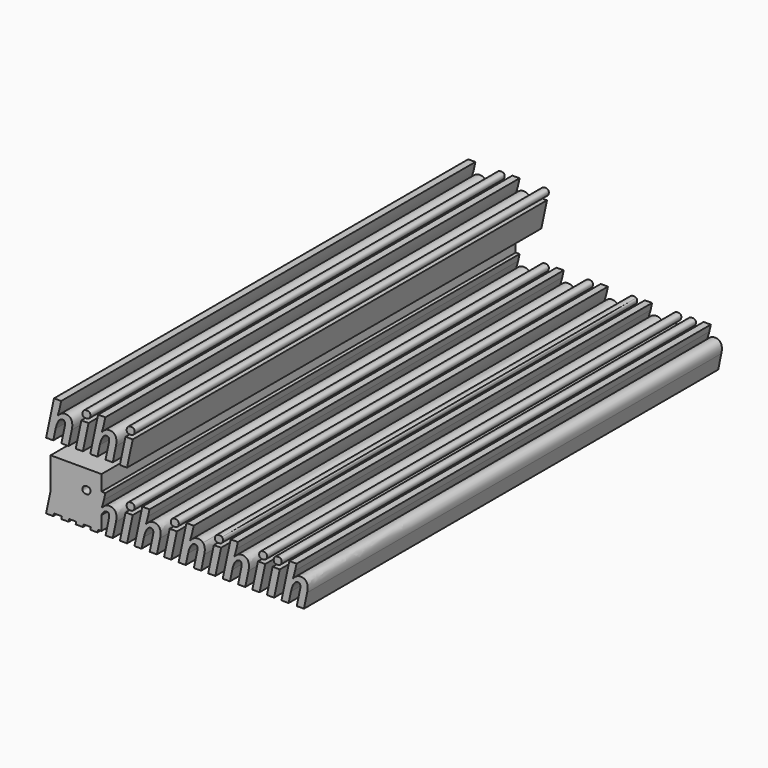
from build123d import *

# Parameters (mm, degrees)
F0_TEXT_SIZE = 47.1805429293
F1_DEPTH     = 498.348


# Not quite as in the source:
# - Text() gives the source's letters only with a copy of the font that has no kerning and outlines rounded to 1/6400 em; it was checked with that copy


with BuildPart() as f1:
    # F0 (on Front) → F1 (new body)
    with BuildSketch(Plane.XZ):
        with BuildLine():
            Line((7.1037112932, -24.0933876485), (14.1806185259, -24.0933876485))
            Line((14.1806185259, -24.0933876485), (21.2442852385, 9.2243729952))
            Line((21.2442852385, 9.2243729952), (24.4913287461, 9.2243729952))
            Line((24.4913287461, 9.2243729952), (24.4913287461, 24.0933876485))
            Line((24.4913287461, 24.0933876485), (-24.4913287461, 24.0933876485))
            Line((-24.4913287461, 24.0933876485), (-24.4913287461, -6.005607145))
            Line((-24.4913287461, -6.005607145), (-21.2624351568, 9.2243729952))
            Line((-21.2624351568, 9.2243729952), (-14.3254209543, 9.2243729952))
            add(Edge.make_bspline(
                [(-14.3254209543, 9.2243729952), (-15.2248000539, 5.0518437298), (-15.7113494028, 2.8181399005)],
                knots=[0, 0, 0, 1, 1, 1], degree=2))
            add(Edge.make_bspline(
                [(-15.7113494028, 2.8181399005), (-16.1978987518, 0.5844360712), (-17.6944065978, -4.3031732979)],
                knots=[0, 0, 0, 1, 1, 1], degree=2))
            Line((-17.6944065978, -4.3031732979), (-17.510107602, -4.3031732979))
            add(Edge.make_bspline(
                [(-17.510107602, -4.3031732979), (-16.0799473944, -2.5265309782), (-14.3291069342, -1.4575968024)],
                knots=[0, 0, 0, 1, 1, 1], degree=2))
            add(Edge.make_bspline(
                [(-14.3291069342, -1.4575968024), (-12.5782664739, -0.3886626267), (-10.2708430463, -0.3886626267)],
                knots=[0, 0, 0, 1, 1, 1], degree=2))
            add(Edge.make_bspline(
                [(-10.2708430463, -0.3886626267), (-7.0935283584, -0.3886626267), (-5.3537458379, -2.3090581631)],
                knots=[0, 0, 0, 1, 1, 1], degree=2))
            add(Edge.make_bspline(
                [(-5.3537458379, -2.3090581631), (-3.6139633173, -4.2294536995), (-3.6139633173, -7.8048542184)],
                knots=[0, 0, 0, 1, 1, 1], degree=2))
            add(Edge.make_bspline(
                [(-3.6139633173, -7.8048542184), (-3.6139633173, -9.4856610603), (-4.1447444253, -11.9478956444)],
                knots=[0, 0, 0, 1, 1, 1], degree=2))
            Line((-4.1447444253, -11.9478956444), (-6.6824263307, -24.0933876485))
            Line((-6.6824263307, -24.0933876485), (0.1733443567, -24.0933876485))
            Line((0.1733443567, -24.0933876485), (5.0923212451, -0.8678400158))
            Line((5.0923212451, -0.8678400158), (12.0293354477, -0.8678400158))
            Line((12.0293354477, -0.8678400158), (7.1037112932, -24.0933876485))
        make_face()
        with BuildLine():
            add(Edge.make_bspline(
                [(9.677680261, 2.3315905516), (6.19811522, 2.3315905516), (6.19811522, 5.1697950872)],
                knots=[0, 0, 0, 1, 1, 1], degree=2))
            add(Edge.make_bspline(
                [(6.19811522, 5.1697950872), (6.19811522, 7.1675962018), (7.2928512551, 8.1959845985)],
                knots=[0, 0, 0, 1, 1, 1], degree=2))
            add(Edge.make_bspline(
                [(7.2928512551, 8.1959845985), (8.3875872903, 9.2243729952), (10.3927603648, 9.2243729952)],
                knots=[0, 0, 0, 1, 1, 1], degree=2))
            add(Edge.make_bspline(
                [(10.3927603648, 9.2243729952), (12.0735672066, 9.2243729952), (12.9508304267, 8.5092928914)],
                knots=[0, 0, 0, 1, 1, 1], degree=2))
            add(Edge.make_bspline(
                [(12.9508304267, 8.5092928914), (13.8280936468, 7.7942127876), (13.8280936468, 6.4598880579)],
                knots=[0, 0, 0, 1, 1, 1], degree=2))
            add(Edge.make_bspline(
                [(13.8280936468, 6.4598880579), (13.8280936468, 4.6168980997), (12.8144491698, 3.4742443256)],
                knots=[0, 0, 0, 1, 1, 1], degree=2))
            add(Edge.make_bspline(
                [(12.8144491698, 3.4742443256), (11.8008046928, 2.3315905516), (9.677680261, 2.3315905516)],
                knots=[0, 0, 0, 1, 1, 1], degree=2))
        make_face(mode=Mode.SUBTRACT)
        with BuildLine():
            Line((21.1106508309, -24.0933876485), (24.4913287461, -24.0933876485))
            Line((24.4913287461, -24.0933876485), (24.4913287461, -10.5974846616))
            add(Edge.make_bspline(
                [(24.4913287461, -10.5974846616), (23.4979536486, -12.8144800029), (22.8366285624, -15.9582417934)],
                knots=[0.3305359837, 0.3305359837, 0.3305359837, 1, 1, 1], degree=2))
            Line((22.8366285624, -15.9582417934), (21.1106508309, -24.0933876485))
        make_face()
        Polygon((20.5734368938, -26.6254676713), (21.1106508309, -24.0933876485), (14.1806185259, -24.0933876485), (13.643794651, -26.6254676713), align=None)
        with BuildLine():
            Line((14.1806185259, -24.0933876485), (21.1106508309, -24.0933876485))
            Line((21.1106508309, -24.0933876485), (22.8366285624, -15.9582417934))
            add(Edge.make_bspline(
                [(24.4913287461, -10.5974846616), (23.4979536486, -12.8144800029), (22.8366285624, -15.9582417934)],
                knots=[0.3305359837, 0.3305359837, 0.3305359837, 1, 1, 1], degree=2))
            Line((24.4913287461, -10.5974846616), (24.4913287461, 9.2243729952))
            Line((24.4913287461, 9.2243729952), (21.2442852385, 9.2243729952))
            Line((21.2442852385, 9.2243729952), (14.1806185259, -24.0933876485))
        make_face()
        with BuildLine():
            Line((24.4913287461, 9.2243729952), (24.4913287461, -10.5974846616))
            add(Edge.make_bspline(
                [(25.5531957607, -8.6341996996), (24.9817900809, -9.5028825349), (24.4913287461, -10.5974846616)],
                knots=[0, 0, 0, 0.3305359837, 0.3305359837, 0.3305359837], degree=2))
            add(Edge.make_bspline(
                [(29.3976728135, -6.0060960192), (27.2819203415, -6.0060960192), (25.5531957607, -8.6341996996)],
                knots=[0, 0, 0, 1, 1, 1], degree=2))
            add(Edge.make_bspline(
                [(31.889395237, -8.836928595), (31.889395237, -6.0060960192), (29.3976728135, -6.0060960192)],
                knots=[0, 0, 0, 1, 1, 1], degree=2))
            add(Edge.make_bspline(
                [(31.5207972453, -11.5792976527), (31.889395237, -10.0164421682), (31.889395237, -8.836928595)],
                knots=[0, 0, 0, 1, 1, 1], degree=2))
            Line((31.5207972453, -11.5792976527), (28.3655984369, -26.6254676713))
            Line((28.3655984369, -26.6254676713), (35.2952406797, -26.6254676713))
            Line((35.2952406797, -26.6254676713), (38.3619759701, -11.9478956444))
            add(Edge.make_bspline(
                [(38.892757078, -7.8048542184), (38.892757078, -9.4856610603), (38.3619759701, -11.9478956444)],
                knots=[0, 0, 0, 1, 1, 1], degree=2))
            add(Edge.make_bspline(
                [(37.1529745575, -2.3090581631), (38.892757078, -4.2294536995), (38.892757078, -7.8048542184)],
                knots=[0, 0, 0, 1, 1, 1], degree=2))
            add(Edge.make_bspline(
                [(32.2358773491, -0.3886626267), (35.413192037, -0.3886626267), (37.1529745575, -2.3090581631)],
                knots=[0, 0, 0, 1, 1, 1], degree=2))
            add(Edge.make_bspline(
                [(28.1776134612, -1.4575968024), (29.9284539215, -0.3886626267), (32.2358773491, -0.3886626267)],
                knots=[0, 0, 0, 1, 1, 1], degree=2))
            add(Edge.make_bspline(
                [(24.9966127934, -4.3031732979), (26.4267730009, -2.5265309782), (28.1776134612, -1.4575968024)],
                knots=[0, 0, 0, 1, 1, 1], degree=2))
            Line((24.9966127934, -4.3031732979), (24.8123137976, -4.3031732979))
            add(Edge.make_bspline(
                [(26.7953709926, 2.8181399005), (26.3088216436, 0.5844360712), (24.8123137976, -4.3031732979)],
                knots=[0, 0, 0, 1, 1, 1], degree=2))
            add(Edge.make_bspline(
                [(28.1812994411, 9.2243729952), (27.2819203415, 5.0518437298), (26.7953709926, 2.8181399005)],
                knots=[0, 0, 0, 1, 1, 1], degree=2))
            Line((28.1812994411, 9.2243729952), (24.4913287461, 9.2243729952))
        make_face()
        Polygon((6.5667132116, -26.6254676713), (7.1037112932, -24.0933876485), (0.1733443567, -24.0933876485), (-0.3629290311, -26.6254676713), align=None)
        Polygon((0.1733443567, -24.0933876485), (7.1037112932, -24.0933876485), (12.0293354477, -0.8678400158), (5.0923212451, -0.8678400158), align=None)
        Polygon((-7.2114797157, -26.6254676713), (-6.6824263307, -24.0933876485), (-13.6101419243, -24.0933876485), (-14.1411219584, -26.6254676713), align=None)
        with BuildLine():
            Line((-13.6101419243, -24.0933876485), (-6.6824263307, -24.0933876485))
            Line((-6.6824263307, -24.0933876485), (-4.1447444253, -11.9478956444))
            add(Edge.make_bspline(
                [(-3.6139633173, -7.8048542184), (-3.6139633173, -9.4856610603), (-4.1447444253, -11.9478956444)],
                knots=[0, 0, 0, 1, 1, 1], degree=2))
            add(Edge.make_bspline(
                [(-5.3537458379, -2.3090581631), (-3.6139633173, -4.2294536995), (-3.6139633173, -7.8048542184)],
                knots=[0, 0, 0, 1, 1, 1], degree=2))
            add(Edge.make_bspline(
                [(-10.2708430463, -0.3886626267), (-7.0935283584, -0.3886626267), (-5.3537458379, -2.3090581631)],
                knots=[0, 0, 0, 1, 1, 1], degree=2))
            add(Edge.make_bspline(
                [(-14.3291069342, -1.4575968024), (-12.5782664739, -0.3886626267), (-10.2708430463, -0.3886626267)],
                knots=[0, 0, 0, 1, 1, 1], degree=2))
            add(Edge.make_bspline(
                [(-17.510107602, -4.3031732979), (-16.0799473944, -2.5265309782), (-14.3291069342, -1.4575968024)],
                knots=[0, 0, 0, 1, 1, 1], degree=2))
            Line((-17.510107602, -4.3031732979), (-17.6944065978, -4.3031732979))
            add(Edge.make_bspline(
                [(-15.7113494028, 2.8181399005), (-16.1978987518, 0.5844360712), (-17.6944065978, -4.3031732979)],
                knots=[0, 0, 0, 1, 1, 1], degree=2))
            add(Edge.make_bspline(
                [(-14.3254209543, 9.2243729952), (-15.2248000539, 5.0518437298), (-15.7113494028, 2.8181399005)],
                knots=[0, 0, 0, 1, 1, 1], degree=2))
            Line((-14.3254209543, 9.2243729952), (-21.2624351568, 9.2243729952))
            Line((-21.2624351568, 9.2243729952), (-24.4913287461, -6.005607145))
            Line((-24.4913287461, -6.005607145), (-24.4913287461, -24.0933876485))
            Line((-24.4913287461, -24.0933876485), (-21.3960695645, -24.0933876485))
            Line((-21.3960695645, -24.0933876485), (-19.670091833, -15.9582417934))
            add(Edge.make_bspline(
                [(-16.9535246346, -8.6341996996), (-18.6822492154, -11.2623033799), (-19.670091833, -15.9582417934)],
                knots=[0, 0, 0, 1, 1, 1], degree=2))
            add(Edge.make_bspline(
                [(-13.1090475819, -6.0060960192), (-15.2248000539, -6.0060960192), (-16.9535246346, -8.6341996996)],
                knots=[0, 0, 0, 1, 1, 1], degree=2))
            add(Edge.make_bspline(
                [(-10.6173251584, -8.836928595), (-10.6173251584, -6.0060960192), (-13.1090475819, -6.0060960192)],
                knots=[0, 0, 0, 1, 1, 1], degree=2))
            add(Edge.make_bspline(
                [(-10.98592315, -11.5792976527), (-10.6173251584, -10.0164421682), (-10.6173251584, -8.836928595)],
                knots=[0, 0, 0, 1, 1, 1], degree=2))
            Line((-10.98592315, -11.5792976527), (-13.6101419243, -24.0933876485))
        make_face()
        Polygon((-24.4913287461, -24.0933876485), (-24.4913287461, -6.005607145), (-28.8629257444, -26.6254676713), (-21.9332835016, -26.6254676713), (-21.3960695645, -24.0933876485), align=None)
        with BuildLine():
            Line((-21.3960695645, -24.0933876485), (-13.6101419243, -24.0933876485))
            Line((-13.6101419243, -24.0933876485), (-10.98592315, -11.5792976527))
            add(Edge.make_bspline(
                [(-10.98592315, -11.5792976527), (-10.6173251584, -10.0164421682), (-10.6173251584, -8.836928595)],
                knots=[0, 0, 0, 1, 1, 1], degree=2))
            add(Edge.make_bspline(
                [(-10.6173251584, -8.836928595), (-10.6173251584, -6.0060960192), (-13.1090475819, -6.0060960192)],
                knots=[0, 0, 0, 1, 1, 1], degree=2))
            add(Edge.make_bspline(
                [(-13.1090475819, -6.0060960192), (-15.2248000539, -6.0060960192), (-16.9535246346, -8.6341996996)],
                knots=[0, 0, 0, 1, 1, 1], degree=2))
            add(Edge.make_bspline(
                [(-16.9535246346, -8.6341996996), (-18.6822492154, -11.2623033799), (-19.670091833, -15.9582417934)],
                knots=[0, 0, 0, 1, 1, 1], degree=2))
            Line((-19.670091833, -15.9582417934), (-21.3960695645, -24.0933876485))
        make_face()
        with Locations((-29.718073085, 37.5400707126)):
            Text('hihi', F0_TEXT_SIZE, font='Open Sans', font_style=FontStyle.BOLDITALIC, text_align=(TextAlign.LEFT, TextAlign.BOTTOM))
        with BuildLine():
            add(Edge.make_bspline(
                [(48.7048356154, 5.1697950872), (48.7048356154, 7.1675962018), (49.7995716505, 8.1959845985)],
                knots=[0, 0, 0, 1, 1, 1], degree=2))
            add(Edge.make_bspline(
                [(52.1844006564, 2.3315905516), (48.7048356154, 2.3315905516), (48.7048356154, 5.1697950872)],
                knots=[0, 0, 0, 1, 1, 1], degree=2))
            add(Edge.make_bspline(
                [(55.3211695652, 3.4742443256), (54.3075250882, 2.3315905516), (52.1844006564, 2.3315905516)],
                knots=[0, 0, 0, 1, 1, 1], degree=2))
            add(Edge.make_bspline(
                [(56.3348140422, 6.4598880579), (56.3348140422, 4.6168980997), (55.3211695652, 3.4742443256)],
                knots=[0, 0, 0, 1, 1, 1], degree=2))
            add(Edge.make_bspline(
                [(55.4575508221, 8.5092928914), (56.3348140422, 7.7942127876), (56.3348140422, 6.4598880579)],
                knots=[0, 0, 0, 1, 1, 1], degree=2))
            add(Edge.make_bspline(
                [(52.8994807602, 9.2243729952), (54.580287602, 9.2243729952), (55.4575508221, 8.5092928914)],
                knots=[0, 0, 0, 1, 1, 1], degree=2))
            add(Edge.make_bspline(
                [(49.7995716505, 8.1959845985), (50.8943076857, 9.2243729952), (52.8994807602, 9.2243729952)],
                knots=[0, 0, 0, 1, 1, 1], degree=2))
        make_face()
        Polygon((42.1437913642, -26.6254676713), (49.073433607, -26.6254676713), (54.536055843, -0.8678400158), (47.5990416404, -0.8678400158), align=None)
        with BuildLine():
            Line((70.8723188323, -26.6254676713), (77.801961075, -26.6254676713))
            Line((77.801961075, -26.6254676713), (80.8686963654, -11.9478956444))
            add(Edge.make_bspline(
                [(81.3994774734, -7.8048542184), (81.3994774734, -9.4856610603), (80.8686963654, -11.9478956444)],
                knots=[0, 0, 0, 1, 1, 1], degree=2))
            add(Edge.make_bspline(
                [(79.6596949529, -2.3090581631), (81.3994774734, -4.2294536995), (81.3994774734, -7.8048542184)],
                knots=[0, 0, 0, 1, 1, 1], degree=2))
            add(Edge.make_bspline(
                [(74.7425977445, -0.3886626267), (77.9199124324, -0.3886626267), (79.6596949529, -2.3090581631)],
                knots=[0, 0, 0, 1, 1, 1], degree=2))
            add(Edge.make_bspline(
                [(70.6843338566, -1.4575968024), (72.4351743168, -0.3886626267), (74.7425977445, -0.3886626267)],
                knots=[0, 0, 0, 1, 1, 1], degree=2))
            add(Edge.make_bspline(
                [(67.5033331887, -4.3031732979), (68.9334933963, -2.5265309782), (70.6843338566, -1.4575968024)],
                knots=[0, 0, 0, 1, 1, 1], degree=2))
            Line((67.5033331887, -4.3031732979), (67.3190341929, -4.3031732979))
            add(Edge.make_bspline(
                [(69.3020913879, 2.8181399005), (68.815542039, 0.5844360712), (67.3190341929, -4.3031732979)],
                knots=[0, 0, 0, 1, 1, 1], degree=2))
            add(Edge.make_bspline(
                [(70.6880198365, 9.2243729952), (69.7886407369, 5.0518437298), (69.3020913879, 2.8181399005)],
                knots=[0, 0, 0, 1, 1, 1], degree=2))
            Line((70.6880198365, 9.2243729952), (63.7510056339, 9.2243729952))
            Line((63.7510056339, 9.2243729952), (56.1505150464, -26.6254676713))
            Line((56.1505150464, -26.6254676713), (63.0801572891, -26.6254676713))
            Line((63.0801572891, -26.6254676713), (65.3433489578, -15.9582417934))
            add(Edge.make_bspline(
                [(68.0599161561, -8.6341996996), (66.3311915753, -11.2623033799), (65.3433489578, -15.9582417934)],
                knots=[0, 0, 0, 1, 1, 1], degree=2))
            add(Edge.make_bspline(
                [(71.9043932089, -6.0060960192), (69.7886407369, -6.0060960192), (68.0599161561, -8.6341996996)],
                knots=[0, 0, 0, 1, 1, 1], degree=2))
            add(Edge.make_bspline(
                [(74.3961156323, -8.836928595), (74.3961156323, -6.0060960192), (71.9043932089, -6.0060960192)],
                knots=[0, 0, 0, 1, 1, 1], degree=2))
            add(Edge.make_bspline(
                [(74.0275176407, -11.5792976527), (74.3961156323, -10.0164421682), (74.3961156323, -8.836928595)],
                knots=[0, 0, 0, 1, 1, 1], degree=2))
            Line((74.0275176407, -11.5792976527), (70.8723188323, -26.6254676713))
        make_face()
        with BuildLine():
            add(Edge.make_bspline(
                [(91.2115560107, 5.1697950872), (91.2115560107, 7.1675962018), (92.3062920459, 8.1959845985)],
                knots=[0, 0, 0, 1, 1, 1], degree=2))
            add(Edge.make_bspline(
                [(94.6911210518, 2.3315905516), (91.2115560107, 2.3315905516), (91.2115560107, 5.1697950872)],
                knots=[0, 0, 0, 1, 1, 1], degree=2))
            add(Edge.make_bspline(
                [(97.8278899606, 3.4742443256), (96.8142454836, 2.3315905516), (94.6911210518, 2.3315905516)],
                knots=[0, 0, 0, 1, 1, 1], degree=2))
            add(Edge.make_bspline(
                [(98.8415344376, 6.4598880579), (98.8415344376, 4.6168980997), (97.8278899606, 3.4742443256)],
                knots=[0, 0, 0, 1, 1, 1], degree=2))
            add(Edge.make_bspline(
                [(97.9642712175, 8.5092928914), (98.8415344376, 7.7942127876), (98.8415344376, 6.4598880579)],
                knots=[0, 0, 0, 1, 1, 1], degree=2))
            add(Edge.make_bspline(
                [(95.4062011555, 9.2243729952), (97.0870079974, 9.2243729952), (97.9642712175, 8.5092928914)],
                knots=[0, 0, 0, 1, 1, 1], degree=2))
            add(Edge.make_bspline(
                [(92.3062920459, 8.1959845985), (93.401028081, 9.2243729952), (95.4062011555, 9.2243729952)],
                knots=[0, 0, 0, 1, 1, 1], degree=2))
        make_face()
        Polygon((84.6505117596, -26.6254676713), (91.5801540024, -26.6254676713), (97.0427762384, -0.8678400158), (90.1057620358, -0.8678400158), align=None)
        with BuildLine():
            Line((113.3790392277, -26.6254676713), (120.3086814704, -26.6254676713))
            Line((120.3086814704, -26.6254676713), (123.3754167608, -11.9478956444))
            add(Edge.make_bspline(
                [(123.9061978688, -7.8048542184), (123.9061978688, -9.4856610603), (123.3754167608, -11.9478956444)],
                knots=[0, 0, 0, 1, 1, 1], degree=2))
            add(Edge.make_bspline(
                [(122.1664153482, -2.3090581631), (123.9061978688, -4.2294536995), (123.9061978688, -7.8048542184)],
                knots=[0, 0, 0, 1, 1, 1], degree=2))
            add(Edge.make_bspline(
                [(117.2493181398, -0.3886626267), (120.4266328277, -0.3886626267), (122.1664153482, -2.3090581631)],
                knots=[0, 0, 0, 1, 1, 1], degree=2))
            add(Edge.make_bspline(
                [(113.1910542519, -1.4575968024), (114.9418947122, -0.3886626267), (117.2493181398, -0.3886626267)],
                knots=[0, 0, 0, 1, 1, 1], degree=2))
            add(Edge.make_bspline(
                [(110.0100535841, -4.3031732979), (111.4402137917, -2.5265309782), (113.1910542519, -1.4575968024)],
                knots=[0, 0, 0, 1, 1, 1], degree=2))
            Line((110.0100535841, -4.3031732979), (109.8257545883, -4.3031732979))
            add(Edge.make_bspline(
                [(111.8088117833, 2.8181399005), (111.3222624343, 0.5844360712), (109.8257545883, -4.3031732979)],
                knots=[0, 0, 0, 1, 1, 1], degree=2))
            add(Edge.make_bspline(
                [(113.1947402318, 9.2243729952), (112.2953611323, 5.0518437298), (111.8088117833, 2.8181399005)],
                knots=[0, 0, 0, 1, 1, 1], degree=2))
            Line((113.1947402318, 9.2243729952), (106.2577260293, 9.2243729952))
            Line((106.2577260293, 9.2243729952), (98.6572354418, -26.6254676713))
            Line((98.6572354418, -26.6254676713), (105.5868776845, -26.6254676713))
            Line((105.5868776845, -26.6254676713), (107.8500693531, -15.9582417934))
            add(Edge.make_bspline(
                [(110.5666365515, -8.6341996996), (108.8379119707, -11.2623033799), (107.8500693531, -15.9582417934)],
                knots=[0, 0, 0, 1, 1, 1], degree=2))
            add(Edge.make_bspline(
                [(114.4111136042, -6.0060960192), (112.2953611323, -6.0060960192), (110.5666365515, -8.6341996996)],
                knots=[0, 0, 0, 1, 1, 1], degree=2))
            add(Edge.make_bspline(
                [(116.9028360277, -8.836928595), (116.9028360277, -6.0060960192), (114.4111136042, -6.0060960192)],
                knots=[0, 0, 0, 1, 1, 1], degree=2))
            add(Edge.make_bspline(
                [(116.5342380361, -11.5792976527), (116.9028360277, -10.0164421682), (116.9028360277, -8.836928595)],
                knots=[0, 0, 0, 1, 1, 1], degree=2))
            Line((116.5342380361, -11.5792976527), (113.3790392277, -26.6254676713))
        make_face()
        with BuildLine():
            add(Edge.make_bspline(
                [(133.7182764061, 5.1697950872), (133.7182764061, 7.1675962018), (134.8130124413, 8.1959845985)],
                knots=[0, 0, 0, 1, 1, 1], degree=2))
            add(Edge.make_bspline(
                [(137.1978414471, 2.3315905516), (133.7182764061, 2.3315905516), (133.7182764061, 5.1697950872)],
                knots=[0, 0, 0, 1, 1, 1], degree=2))
            add(Edge.make_bspline(
                [(140.3346103559, 3.4742443256), (139.320965879, 2.3315905516), (137.1978414471, 2.3315905516)],
                knots=[0, 0, 0, 1, 1, 1], degree=2))
            add(Edge.make_bspline(
                [(141.3482548329, 6.4598880579), (141.3482548329, 4.6168980997), (140.3346103559, 3.4742443256)],
                knots=[0, 0, 0, 1, 1, 1], degree=2))
            add(Edge.make_bspline(
                [(140.4709916129, 8.5092928914), (141.3482548329, 7.7942127876), (141.3482548329, 6.4598880579)],
                knots=[0, 0, 0, 1, 1, 1], degree=2))
            add(Edge.make_bspline(
                [(137.9129215509, 9.2243729952), (139.5937283928, 9.2243729952), (140.4709916129, 8.5092928914)],
                knots=[0, 0, 0, 1, 1, 1], degree=2))
            add(Edge.make_bspline(
                [(134.8130124413, 8.1959845985), (135.9077484764, 9.2243729952), (137.9129215509, 9.2243729952)],
                knots=[0, 0, 0, 1, 1, 1], degree=2))
        make_face()
        Polygon((127.157232155, -26.6254676713), (134.0868743977, -26.6254676713), (139.5494966338, -0.8678400158), (132.6124824312, -0.8678400158), align=None)
        with BuildLine():
            Line((155.885759623, -26.6254676713), (162.8154018658, -26.6254676713))
            Line((162.8154018658, -26.6254676713), (165.8821371562, -11.9478956444))
            add(Edge.make_bspline(
                [(166.4129182641, -7.8048542184), (166.4129182641, -9.4856610603), (165.8821371562, -11.9478956444)],
                knots=[0, 0, 0, 1, 1, 1], degree=2))
            add(Edge.make_bspline(
                [(164.6731357436, -2.3090581631), (166.4129182641, -4.2294536995), (166.4129182641, -7.8048542184)],
                knots=[0, 0, 0, 1, 1, 1], degree=2))
            add(Edge.make_bspline(
                [(159.7560385352, -0.3886626267), (162.9333532231, -0.3886626267), (164.6731357436, -2.3090581631)],
                knots=[0, 0, 0, 1, 1, 1], degree=2))
            add(Edge.make_bspline(
                [(155.6977746473, -1.4575968024), (157.4486151076, -0.3886626267), (159.7560385352, -0.3886626267)],
                knots=[0, 0, 0, 1, 1, 1], degree=2))
            add(Edge.make_bspline(
                [(152.5167739795, -4.3031732979), (153.946934187, -2.5265309782), (155.6977746473, -1.4575968024)],
                knots=[0, 0, 0, 1, 1, 1], degree=2))
            Line((152.5167739795, -4.3031732979), (152.3324749837, -4.3031732979))
            add(Edge.make_bspline(
                [(154.3155321787, 2.8181399005), (153.8289828297, 0.5844360712), (152.3324749837, -4.3031732979)],
                knots=[0, 0, 0, 1, 1, 1], degree=2))
            add(Edge.make_bspline(
                [(155.7014606272, 9.2243729952), (154.8020815276, 5.0518437298), (154.3155321787, 2.8181399005)],
                knots=[0, 0, 0, 1, 1, 1], degree=2))
            Line((155.7014606272, 9.2243729952), (148.7644464246, 9.2243729952))
            Line((148.7644464246, 9.2243729952), (141.1639558371, -26.6254676713))
            Line((141.1639558371, -26.6254676713), (148.0935980799, -26.6254676713))
            Line((148.0935980799, -26.6254676713), (150.3567897485, -15.9582417934))
            add(Edge.make_bspline(
                [(153.0733569469, -8.6341996996), (151.3446323661, -11.2623033799), (150.3567897485, -15.9582417934)],
                knots=[0, 0, 0, 1, 1, 1], degree=2))
            add(Edge.make_bspline(
                [(156.9178339996, -6.0060960192), (154.8020815276, -6.0060960192), (153.0733569469, -8.6341996996)],
                knots=[0, 0, 0, 1, 1, 1], degree=2))
            add(Edge.make_bspline(
                [(159.4095564231, -8.836928595), (159.4095564231, -6.0060960192), (156.9178339996, -6.0060960192)],
                knots=[0, 0, 0, 1, 1, 1], degree=2))
            add(Edge.make_bspline(
                [(159.0409584314, -11.5792976527), (159.4095564231, -10.0164421682), (159.4095564231, -8.836928595)],
                knots=[0, 0, 0, 1, 1, 1], degree=2))
            Line((159.0409584314, -11.5792976527), (155.885759623, -26.6254676713))
        make_face()
        with BuildLine():
            add(Edge.make_bspline(
                [(176.2249968015, 5.1697950872), (176.2249968015, 7.1675962018), (177.3197328366, 8.1959845985)],
                knots=[0, 0, 0, 1, 1, 1], degree=2))
            add(Edge.make_bspline(
                [(179.7045618425, 2.3315905516), (176.2249968015, 2.3315905516), (176.2249968015, 5.1697950872)],
                knots=[0, 0, 0, 1, 1, 1], degree=2))
            add(Edge.make_bspline(
                [(182.8413307513, 3.4742443256), (181.8276862743, 2.3315905516), (179.7045618425, 2.3315905516)],
                knots=[0, 0, 0, 1, 1, 1], degree=2))
            add(Edge.make_bspline(
                [(183.8549752283, 6.4598880579), (183.8549752283, 4.6168980997), (182.8413307513, 3.4742443256)],
                knots=[0, 0, 0, 1, 1, 1], degree=2))
            add(Edge.make_bspline(
                [(182.9777120082, 8.5092928914), (183.8549752283, 7.7942127876), (183.8549752283, 6.4598880579)],
                knots=[0, 0, 0, 1, 1, 1], degree=2))
            add(Edge.make_bspline(
                [(180.4196419463, 9.2243729952), (182.1004487881, 9.2243729952), (182.9777120082, 8.5092928914)],
                knots=[0, 0, 0, 1, 1, 1], degree=2))
            add(Edge.make_bspline(
                [(177.3197328366, 8.1959845985), (178.4144688718, 9.2243729952), (180.4196419463, 9.2243729952)],
                knots=[0, 0, 0, 1, 1, 1], degree=2))
        make_face()
        Polygon((169.6639525504, -26.6254676713), (176.5935947931, -26.6254676713), (182.0562170291, -0.8678400158), (175.1192028266, -0.8678400158), align=None)
        with BuildLine():
            add(Edge.make_bspline(
                [(190.2317204836, 5.1697950872), (190.2317204836, 7.1675962018), (191.3264565188, 8.1959845985)],
                knots=[0, 0, 0, 1, 1, 1], degree=2))
            add(Edge.make_bspline(
                [(193.7112855246, 2.3315905516), (190.2317204836, 2.3315905516), (190.2317204836, 5.1697950872)],
                knots=[0, 0, 0, 1, 1, 1], degree=2))
            add(Edge.make_bspline(
                [(196.8480544335, 3.4742443256), (195.8344099565, 2.3315905516), (193.7112855246, 2.3315905516)],
                knots=[0, 0, 0, 1, 1, 1], degree=2))
            add(Edge.make_bspline(
                [(197.8616989105, 6.4598880579), (197.8616989105, 4.6168980997), (196.8480544335, 3.4742443256)],
                knots=[0, 0, 0, 1, 1, 1], degree=2))
            add(Edge.make_bspline(
                [(196.9844356904, 8.5092928914), (197.8616989105, 7.7942127876), (197.8616989105, 6.4598880579)],
                knots=[0, 0, 0, 1, 1, 1], degree=2))
            add(Edge.make_bspline(
                [(194.4263656284, 9.2243729952), (196.1071724703, 9.2243729952), (196.9844356904, 8.5092928914)],
                knots=[0, 0, 0, 1, 1, 1], degree=2))
            add(Edge.make_bspline(
                [(191.3264565188, 8.1959845985), (192.4211925539, 9.2243729952), (194.4263656284, 9.2243729952)],
                knots=[0, 0, 0, 1, 1, 1], degree=2))
        make_face()
        Polygon((183.6706762325, -26.6254676713), (190.6003184752, -26.6254676713), (196.0629407113, -0.8678400158), (189.1259265087, -0.8678400158), align=None)
        with BuildLine():
            Line((212.3992037005, -26.6254676713), (219.3288459433, -26.6254676713))
            Line((219.3288459433, -26.6254676713), (222.3955812337, -11.9478956444))
            add(Edge.make_bspline(
                [(222.9263623416, -7.8048542184), (222.9263623416, -9.4856610603), (222.3955812337, -11.9478956444)],
                knots=[0, 0, 0, 1, 1, 1], degree=2))
            add(Edge.make_bspline(
                [(221.1865798211, -2.3090581631), (222.9263623416, -4.2294536995), (222.9263623416, -7.8048542184)],
                knots=[0, 0, 0, 1, 1, 1], degree=2))
            add(Edge.make_bspline(
                [(216.2694826127, -0.3886626267), (219.4467973006, -0.3886626267), (221.1865798211, -2.3090581631)],
                knots=[0, 0, 0, 1, 1, 1], degree=2))
            add(Edge.make_bspline(
                [(212.2112187248, -1.4575968024), (213.9620591851, -0.3886626267), (216.2694826127, -0.3886626267)],
                knots=[0, 0, 0, 1, 1, 1], degree=2))
            add(Edge.make_bspline(
                [(209.030218057, -4.3031732979), (210.4603782645, -2.5265309782), (212.2112187248, -1.4575968024)],
                knots=[0, 0, 0, 1, 1, 1], degree=2))
            Line((209.030218057, -4.3031732979), (208.8459190612, -4.3031732979))
            add(Edge.make_bspline(
                [(210.8289762562, 2.8181399005), (210.3424269072, 0.5844360712), (208.8459190612, -4.3031732979)],
                knots=[0, 0, 0, 1, 1, 1], degree=2))
            add(Edge.make_bspline(
                [(212.2149047047, 9.2243729952), (211.3155256051, 5.0518437298), (210.8289762562, 2.8181399005)],
                knots=[0, 0, 0, 1, 1, 1], degree=2))
            Line((212.2149047047, 9.2243729952), (205.2778905022, 9.2243729952))
            Line((205.2778905022, 9.2243729952), (197.6773999146, -26.6254676713))
            Line((197.6773999146, -26.6254676713), (204.6070421574, -26.6254676713))
            Line((204.6070421574, -26.6254676713), (206.870233826, -15.9582417934))
            add(Edge.make_bspline(
                [(209.5868010244, -8.6341996996), (207.8580764436, -11.2623033799), (206.870233826, -15.9582417934)],
                knots=[0, 0, 0, 1, 1, 1], degree=2))
            add(Edge.make_bspline(
                [(213.4312780771, -6.0060960192), (211.3155256051, -6.0060960192), (209.5868010244, -8.6341996996)],
                knots=[0, 0, 0, 1, 1, 1], degree=2))
            add(Edge.make_bspline(
                [(215.9230005006, -8.836928595), (215.9230005006, -6.0060960192), (213.4312780771, -6.0060960192)],
                knots=[0, 0, 0, 1, 1, 1], degree=2))
            add(Edge.make_bspline(
                [(215.5544025089, -11.5792976527), (215.9230005006, -10.0164421682), (215.9230005006, -8.836928595)],
                knots=[0, 0, 0, 1, 1, 1], degree=2))
            Line((215.5544025089, -11.5792976527), (212.3992037005, -26.6254676713))
        make_face()
    extrude(amount=F1_DEPTH)


solid = f1.part
